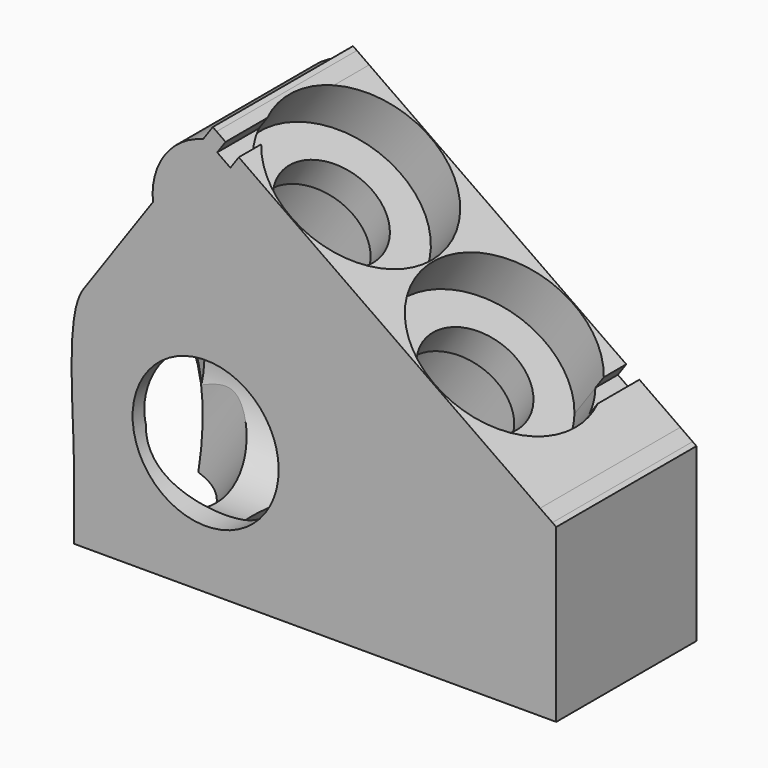
from build123d import *

# Parameters (mm, degrees)
F1_DEPTH  = 6
F2_R      = 5
F3_DEPTH  = 25
F5_START  = -5.8
F4_R      = 5
F4_R_2    = 3.5
F5_DEPTH  = 26.5
F6_DEPTH  = 38.4
F7_DEPTH  = 3.5
F8_R      = 5.1455726412
F9_DEPTH  = 22.6
F10_DEPTH = 1


with BuildPart() as f1:
    # F0 (on Front) → F1 (new body, symmetric)
    with BuildSketch(Plane.XZ):
        Polygon((-15.9628038305, 4), (-7.0709644092, 4), (-5.1744842522, 6.7084543561), (-1.7330256341, 11.6233666218), (-1.1058552598, 12.5190587418), (-22.4038084113, 27.4320460869), (-23.0309787856, 26.5363539669), (-26.4724374037, 21.6214417012), (-31.2942431747, 14.7351894004), align=None)
        Polygon((-25.9186847038, 24.76593569), (-26.4724374037, 21.6214417012), (-23.0309787856, 26.5363539669), (-25.2341914491, 25.1855903927), align=None)
        Polygon((-32.4000984345, 15.5095175895), (-31.2942431747, 14.7351894004), (-26.4724374037, 21.6214417012), (-25.9186847038, 24.76593569), (-27.6068595339, 22.3549721713), align=None)
        with BuildLine():
            ThreePointArc((-24.1761827572, 27.2544863717), (-26.8028128996, 25.4428226271), (-27.6068595339, 22.3549721713))
            Line((-27.6068595339, 22.3549721713), (-25.9186847038, 24.76593569))
            Line((-25.9186847038, 24.76593569), (-24.1761827572, 27.2544863717))
        make_face()
        Polygon((-25.2341914491, 25.1855903927), (-23.0309787856, 26.5363539669), (-22.4038084113, 27.4320460869), (-23.2475350169, 28.0228298164), align=None)
        Polygon((-24.1761827572, 27.2544863717), (-25.9186847038, 24.76593569), (-25.2341914491, 25.1855903927), (-23.2475350169, 28.0228298164), (-23.5096636711, 28.206374276), align=None)
        with BuildLine():
            Line((-33, 4), (-15.9628038305, 4))
            Line((-15.9628038305, 4), (-31.2942431747, 14.7351894004))
            Line((-31.2942431747, 14.7351894004), (-32.4000984345, 15.5095175895))
            add(Edge.make_bspline(
                [(-32.4000984345, 15.5095175895), (-33.6793400347, 13.5531779379), (-33, 7.9824011773), (-33, 4)],
                knots=[0, 0, 0, 0, 11.5251410851, 11.5251410851, 11.5251410851, 11.5251410851], degree=3))
        make_face()
        Polygon((-33, 0), (-10.2502118035, 0), (-15.9628038305, 4), (-33, 4), align=None)
        Polygon((-10.2502118035, 0), (-9.8717945621, 0), (-7.0709644092, 4), (-15.9628038305, 4), align=None)
        Polygon((-9.8717945621, 0), (0, 0), (0, 4), (-7.0709644092, 4), align=None)
        Polygon((-7.0709644092, 4), (0, 4), (0, 7.8723652764), (0, 11.7447305527), (-0.2621286542, 11.9282750123), (-2.2487850863, 9.0910355887), (-2.4090210327, 8.3042919667), (-5.1744842522, 6.7084543561), align=None)
        Polygon((-1.7330256341, 11.6233666218), (-5.1744842522, 6.7084543561), (-2.4090210327, 8.3042919667), (-2.2487850863, 9.0910355887), align=None)
        Polygon((-1.1058552598, 12.5190587418), (-1.7330256341, 11.6233666218), (-2.2487850863, 9.0910355887), (-0.2621286542, 11.9282750123), align=None)
    extrude(amount=F1_DEPTH, both=True)

    # F2 (on face) → F3 (cut)
    with BuildSketch(Plane.XZ.offset(6)):
        with Locations((-24, 9)):
            Circle(F2_R)
    extrude(amount=-F3_DEPTH, mode=Mode.SUBTRACT)

    # F4 (on face) → F5 (cut)
    with BuildSketch(Plane(origin=(5.5182183168, 0, 7.8808324898), x_dir=(0.8191520443, 0, -0.5735764364), z_dir=(0.5735764364, 0, 0.8191520443)).offset(F5_START)):
        with Locations((-28.9365006963, 0)):
            Circle(F4_R)
        with Locations((-28.9365006963, 0)):
            Circle(F4_R_2, mode=Mode.SUBTRACT)
        with Locations((-16.9365006963, 0)):
            Circle(F4_R)
        with Locations((-16.9365006963, 0)):
            Circle(F4_R_2, mode=Mode.SUBTRACT)
    extrude(amount=-F5_DEPTH, mode=Mode.SUBTRACT)

    # F4 (on face) → F6 (cut)
    with BuildSketch(Plane(origin=(5.5182183168, 0, 7.8808324898), x_dir=(0.8191520443, 0, -0.5735764364), z_dir=(0.5735764364, 0, 0.8191520443))):
        with Locations((-28.9365006963, 0)):
            Circle(F4_R_2)
        with Locations((-16.9365006963, 0)):
            Circle(F4_R_2)
    extrude(amount=-F6_DEPTH, mode=Mode.SUBTRACT)

    # F4 (on face) → F7 (cut)
    with BuildSketch(Plane(origin=(5.5182183168, 0, 7.8808324898), x_dir=(0.8191520443, 0, -0.5735764364), z_dir=(0.5735764364, 0, 0.8191520443))):
        with BuildLine():
            ThreePointArc((-33.2675799668, -4.0797367995), (-26.7418961373, -5.5304801627), (-22.9865006963, 0))
            ThreePointArc((-22.9865006963, 0), (-30.1789938232, 5.8188238356), (-34.3675799668, -2.4302012176))
            ThreePointArc((-34.3675799668, -2.4302012176), (-33.8867710681, -3.3011093963), (-33.2675799668, -4.0797367995))
        make_face()
        with Locations((-28.9365006963, 0)):
            Circle(F4_R, mode=Mode.SUBTRACT)
        with BuildLine():
            ThreePointArc((-11.5054206963, 2.4301995872), (-11.9862295339, 3.3011082107), (-12.6054206963, 4.079736025))
            ThreePointArc((-12.6054206963, 4.079736025), (-22.4669810552, -2.1946040645), (-10.9865006963, 0))
            ThreePointArc((-10.9865006963, 0), (-11.1176766742, 1.2424922535), (-11.5054206963, 2.4301995872))
        make_face()
        with Locations((-16.9365006963, 0)):
            Circle(F4_R, mode=Mode.SUBTRACT)
        with Locations((-28.9365006963, 0)):
            Circle(F4_R)
        with Locations((-28.9365006963, 0)):
            Circle(F4_R_2, mode=Mode.SUBTRACT)
        with Locations((-16.9365006963, 0)):
            Circle(F4_R)
        with Locations((-16.9365006963, 0)):
            Circle(F4_R_2, mode=Mode.SUBTRACT)
    extrude(amount=-F7_DEPTH, mode=Mode.SUBTRACT)

    # F8 (on face) → F9 (cut)
    with BuildSketch(Plane(origin=(-33, 0, 0), x_dir=(0, -1, 0), z_dir=(-1, 0, 0))):
        with Locations((0, 6.7609399557)):
            Circle(F8_R)
    extrude(amount=-F9_DEPTH, mode=Mode.SUBTRACT)

    # F4 (on face) → F10 (cut)
    with BuildSketch(Plane(origin=(5.5182183168, 0, 7.8808324898), x_dir=(0.8191520443, 0, -0.5735764364), z_dir=(0.5735764364, 0, 0.8191520443))):
        with BuildLine():
            ThreePointArc((-33.2675799668, -4.0797367995), (-33.8867710681, -3.3011093963), (-34.3675799668, -2.4302012176))
            Line((-34.3675799668, -2.4302012176), (-34.3675799668, -6))
            Line((-34.3675799668, -6), (-33.2675799668, -6))
            Line((-33.2675799668, -6), (-33.2675799668, -4.0797367995))
        make_face()
        with BuildLine():
            Line((-11.5054206963, 6), (-12.6054206963, 6))
            Line((-12.6054206963, 6), (-12.6054206963, 4.079736025))
            ThreePointArc((-12.6054206963, 4.079736025), (-11.9862295339, 3.3011082107), (-11.5054206963, 2.4301995872))
            Line((-11.5054206963, 2.4301995872), (-11.5054206963, 6))
        make_face()
    extrude(amount=-F10_DEPTH, mode=Mode.SUBTRACT)


solid = f1.part
